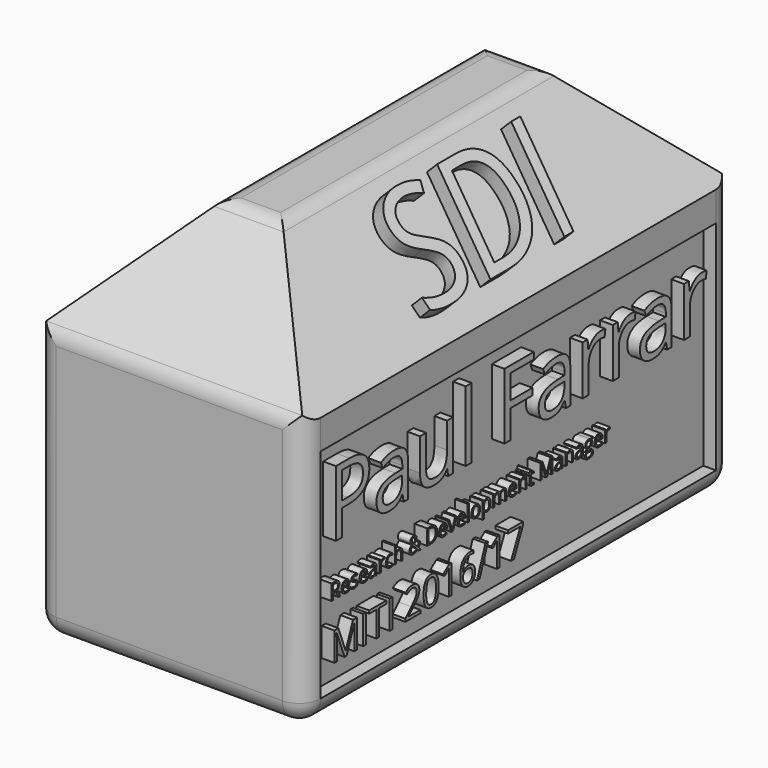
from build123d import *

# Parameters (mm, degrees)
F0_W                    = 63.5
F0_H                    = 63.5
F1_DEPTH                = 63.5
F1_DEPTH_BACK           = 63.5
F2_W                    = 63.5
F2_H                    = 127
F3_DEPTH                = 25
F3_TAPER                = 45
F4_TEXT_SIZE            = 32.8258540119
F5_DEPTH                = 3.4
F6_W                    = 117
F6_H                    = 51.5
F7_DEPTH                = 3
F8_TEXT_SIZE            = 21.8211226941
F8_TEXT_SIZE_2          = 5.1185339948
F8_TEXT_SIZE_3          = 9.4288791944
F9_DEPTH                = 3
F10_W                   = 43.5
F10_H                   = 107
F11_DEPTH               = 60
F12_R                   = 10
F13_R                   = 5
F14_T1_DEPTH            = 53.5
F14_T3_DEPTH            = 71
F14_T5_DEPTH            = 73.8553390593
F14_T7_DEPTH            = 117
F14_T9_DEPTH            = 87.3553390593
F14_T11_DEPTH           = 23.8553390593
F14_S15_W               = 5
F14_S15_H               = 5
F14_T16_DEPTH           = 5
F14_S21_W               = 5
F14_S21_H               = 5
F14_T22_DEPTH           = 5
F14_S27_W               = 5
F14_S27_H               = 5
F14_T28_DEPTH           = 5
F14_S33_W               = 5
F14_S33_H               = 5
F14_T34_DEPTH           = 5
F15_W                   = 33.5
F15_H                   = 87
F16_DEPTH               = 23.2
DRAFT_F16_DRAFTED_ANGLE = 25
F17_R                   = 5


# Not quite as in the source:
# - a fillet or chamfer that OpenCascade refuses, or shapes differently, is made with other operations: its cross-section is extruded or revolved along the edge and cut away or added
# - an extrude with a draft is written as a straight extrude whose walls are then drafted
# - Text() gives the source's letters only with a copy of the font that has no kerning and outlines rounded to 1/6400 em; it was checked with that copy


with BuildPart() as f1:
    # F0 (on Front) → F1 (new body, two sides)
    with BuildSketch(Plane.XZ) as f1_sk:
        Rectangle(F0_W, F0_H)
    extrude(amount=-F1_DEPTH)
    extrude(f1_sk.sketch, amount=F1_DEPTH_BACK)

    # F2 (on face) → F3 (join)
    with BuildSketch(Plane.XY.offset(31.75)):
        Rectangle(F2_W, F2_H)
    extrude(amount=F3_DEPTH, taper=F3_TAPER)

    # F4 (on face) → F5 (join)
    with BuildSketch(Plane(origin=(31.75, 0, 31.75), x_dir=(0, 1, 0), z_dir=(0.7071067812, 0, 0.7071067812))):
        with Locations((-23.613194935, 6.1781886034)):
            Text('SDI', F4_TEXT_SIZE, font='Open Sans', font_style=FontStyle.ITALIC, text_align=(TextAlign.LEFT, TextAlign.BOTTOM))
    extrude(amount=F5_DEPTH)

    # F6 (on face) → F7 (cut)
    with BuildSketch(Plane.YZ.offset(31.75)):
        with Locations((0, -1)):
            Rectangle(F6_W, F6_H)
    extrude(amount=-F7_DEPTH, mode=Mode.SUBTRACT)

    # F8 (on face) → F9 (join)
    with BuildSketch(Plane.YZ.offset(28.75)):
        with Locations((-56.0560356826, 4.2672422715)):
            Text('Paul Farrar', F8_TEXT_SIZE, font='Open Sans', text_align=(TextAlign.LEFT, TextAlign.BOTTOM))
        with Locations((-55.66810444, -7.7586206608)):
            Text('Research & Development Manager', F8_TEXT_SIZE_2, font='Open Sans', text_align=(TextAlign.LEFT, TextAlign.BOTTOM))
        with Locations((-55.28017506, -20.9482768551)):
            Text('MITI 2016/17', F8_TEXT_SIZE_3, font='Open Sans', text_align=(TextAlign.LEFT, TextAlign.BOTTOM))
    extrude(amount=F9_DEPTH)

    # F10 (on face) → F11 (cut)
    with BuildSketch(Plane(origin=(0, 0, -31.75), x_dir=(1, 0, 0), z_dir=(0, 0, -1))):
        Rectangle(F10_W, F10_H)
    extrude(amount=-F11_DEPTH, mode=Mode.SUBTRACT)

    # F12
    f12_edges = [f1.edges().sort_by_distance(p)[0] for p in [
        (0, -53.5, 28.25),
        (0, 53.5, 28.25),
    ]]
    fillet(f12_edges, radius=F12_R)

    # F13
    f13_edges = [f1.edges().sort_by_distance(p)[0] for p in [
        (21.75, 0, 28.25),
        (-21.75, 0, 28.25),
    ]]
    fillet(f13_edges, radius=F13_R)

    # F14: fillet of radius 5 on 14 edges, made by hand

    # F14_s2 → F14_t1 (cut)
    with BuildSketch(Plane.YZ.offset(-26.75)):
        with BuildLine():
            ThreePointArc((58.5, -31.75), (62.0355339059, -30.2855339059), (63.5, -26.75))
            Line((63.5, -26.75), (63.5, -31.75))
            Line((63.5, -31.75), (58.5, -31.75))
        make_face()
        with BuildLine():
            ThreePointArc((-58.5, -31.75), (-62.0355339059, -30.2855339059), (-63.5, -26.75))
            Line((-63.5, -26.75), (-63.5, -31.75))
            Line((-63.5, -31.75), (-58.5, -31.75))
        make_face()
    extrude(amount=F14_T1_DEPTH, mode=Mode.SUBTRACT)

    # F14_s4 → F14_t3 (cut)
    with BuildSketch(Plane.XY.offset(-26.75)):
        with BuildLine():
            ThreePointArc((26.75, 63.5), (30.2855339059, 62.0355339059), (31.75, 58.5))
            Line((31.75, 58.5), (31.75, 63.5))
            Line((31.75, 63.5), (26.75, 63.5))
        make_face()
        with BuildLine():
            ThreePointArc((-26.75, 63.5), (-30.2855339059, 62.0355339059), (-31.75, 58.5))
            Line((-31.75, 58.5), (-31.75, 63.5))
            Line((-31.75, 63.5), (-26.75, 63.5))
        make_face()
        with BuildLine():
            ThreePointArc((31.75, -58.5), (30.2855339059, -62.0355339059), (26.75, -63.5))
            Line((26.75, -63.5), (31.75, -63.5))
            Line((31.75, -63.5), (31.75, -58.5))
        make_face()
        with BuildLine():
            ThreePointArc((-31.75, -58.5), (-30.2855339059, -62.0355339059), (-26.75, -63.5))
            Line((-26.75, -63.5), (-31.75, -63.5))
            Line((-31.75, -63.5), (-31.75, -58.5))
        make_face()
    extrude(amount=F14_T3_DEPTH, mode=Mode.SUBTRACT)

    # F14_s6 → F14_t5 (cut)
    with BuildSketch(Plane.YZ.offset(-36.9276695297)):
        with BuildLine():
            ThreePointArc((63.5, 29.6789321881), (63.1193976626, 31.59234935), (62.0355339059, 33.2144660941))
            Line((62.0355339059, 33.2144660941), (63.5, 31.75))
            Line((63.5, 31.75), (63.5, 29.6789321881))
        make_face()
        with BuildLine():
            ThreePointArc((-63.5, 29.6789321881), (-63.1193976626, 31.59234935), (-62.0355339059, 33.2144660941))
            Line((-62.0355339059, 33.2144660941), (-63.5, 31.75))
            Line((-63.5, 31.75), (-63.5, 29.6789321881))
        make_face()
    extrude(amount=F14_T5_DEPTH, mode=Mode.SUBTRACT)

    # F14_s8 → F14_t7 (cut)
    with BuildSketch(Plane.XZ.offset(-58.5)):
        with BuildLine():
            ThreePointArc((-26.75, -31.75), (-30.2855339059, -30.2855339059), (-31.75, -26.75))
            Line((-31.75, -26.75), (-31.75, -31.75))
            Line((-31.75, -31.75), (-26.75, -31.75))
        make_face()
        with BuildLine():
            ThreePointArc((26.75, -31.75), (30.2855339059, -30.2855339059), (31.75, -26.75))
            Line((31.75, -26.75), (31.75, -31.75))
            Line((31.75, -31.75), (26.75, -31.75))
        make_face()
    extrude(amount=F14_T7_DEPTH, mode=Mode.SUBTRACT)

    # F14_s10 → F14_t9 (cut)
    with BuildSketch(Plane.XZ.offset(-43.6776695297)):
        with BuildLine():
            ThreePointArc((8.2144660941, 55.2855339059), (6.59234935, 56.3693976626), (4.6789321881, 56.75))
            Line((4.6789321881, 56.75), (6.75, 56.75))
            Line((6.75, 56.75), (8.2144660941, 55.2855339059))
        make_face()
        with BuildLine():
            ThreePointArc((-8.2144660941, 55.2855339059), (-6.59234935, 56.3693976626), (-4.6789321881, 56.75))
            Line((-4.6789321881, 56.75), (-6.75, 56.75))
            Line((-6.75, 56.75), (-8.2144660941, 55.2855339059))
        make_face()
    extrude(amount=F14_T9_DEPTH, mode=Mode.SUBTRACT)

    # F14_s12 → F14_t11 (cut)
    with BuildSketch(Plane.YZ.offset(-11.9276695297)):
        with BuildLine():
            ThreePointArc((39.9644660941, 55.2855339059), (38.34234935, 56.3693976626), (36.4289321881, 56.75))
            Line((36.4289321881, 56.75), (38.5, 56.75))
            Line((38.5, 56.75), (39.9644660941, 55.2855339059))
        make_face()
        with BuildLine():
            ThreePointArc((-39.9644660941, 55.2855339059), (-38.34234935, 56.3693976626), (-36.4289321881, 56.75))
            Line((-36.4289321881, 56.75), (-38.5, 56.75))
            Line((-38.5, 56.75), (-39.9644660941, 55.2855339059))
        make_face()
    extrude(amount=F14_T11_DEPTH, mode=Mode.SUBTRACT)


with BuildPart() as f14_tool14:
    # F14_s15 → F14_t16 (new body)
    with BuildSketch(Plane.XY.offset(-26.75)):
        with Locations((-29.25, 61)):
            Rectangle(F14_S15_W, F14_S15_H)
    extrude(amount=-F14_T16_DEPTH)

    # F14_s17 → F14_t18 (revolve, cut)
    with BuildSketch(Plane(origin=(-26.75, 58.5, -26.75), x_dir=(0.7071067812, -0.7071067812, 0), z_dir=(0.7071067812, 0.7071067812, 0))):
        with BuildLine():
            ThreePointArc((0, -5), (5, 0), (0, 5))
            Line((0, 5), (0, -5))
        make_face()
    revolve(axis=Axis((-26.75, 58.5, -26.75), (0, 0, -1)), mode=Mode.SUBTRACT)


with BuildPart() as f1_1:
    add(f1.part)

    # F14_t13: cut F14_tool14
    add(f14_tool14.part, mode=Mode.SUBTRACT)


with BuildPart() as f14_tool20:
    # F14_s21 → F14_t22 (new body)
    with BuildSketch(Plane.XY.offset(-26.75)):
        with Locations((29.25, 61)):
            Rectangle(F14_S21_W, F14_S21_H)
    extrude(amount=-F14_T22_DEPTH)

    # F14_s23 → F14_t24 (revolve, cut)
    with BuildSketch(Plane(origin=(26.75, 58.5, -26.75), x_dir=(-0.7071067812, -0.7071067812, 0), z_dir=(0.7071067812, -0.7071067812, 0))):
        with BuildLine():
            ThreePointArc((0, -5), (5, 0), (0, 5))
            Line((0, 5), (0, -5))
        make_face()
    revolve(axis=Axis((26.75, 58.5, -26.75), (0, 0, -1)), mode=Mode.SUBTRACT)


with BuildPart() as f1_2:
    add(f1_1.part)

    # F14_t19: cut F14_tool20
    add(f14_tool20.part, mode=Mode.SUBTRACT)


with BuildPart() as f14_tool26:
    # F14_s27 → F14_t28 (new body)
    with BuildSketch(Plane.XY.offset(-26.75)):
        with Locations((-29.25, -61)):
            Rectangle(F14_S27_W, F14_S27_H)
    extrude(amount=-F14_T28_DEPTH)

    # F14_s29 → F14_t30 (revolve, cut)
    with BuildSketch(Plane(origin=(-26.75, -58.5, -26.75), x_dir=(0.7071067812, 0.7071067812, 0), z_dir=(-0.7071067812, 0.7071067812, 0))):
        with BuildLine():
            ThreePointArc((0, -5), (5, 0), (0, 5))
            Line((0, 5), (0, -5))
        make_face()
    revolve(axis=Axis((-26.75, -58.5, -26.75), (0, 0, -1)), mode=Mode.SUBTRACT)


with BuildPart() as f1_3:
    add(f1_2.part)

    # F14_t25: cut F14_tool26
    add(f14_tool26.part, mode=Mode.SUBTRACT)


with BuildPart() as f14_tool32:
    # F14_s33 → F14_t34 (new body)
    with BuildSketch(Plane.XY.offset(-26.75)):
        with Locations((29.25, -61)):
            Rectangle(F14_S33_W, F14_S33_H)
    extrude(amount=-F14_T34_DEPTH)

    # F14_s35 → F14_t36 (revolve, cut)
    with BuildSketch(Plane(origin=(26.75, -58.5, -26.75), x_dir=(-0.7071067812, 0.7071067812, 0), z_dir=(-0.7071067812, -0.7071067812, 0))):
        with BuildLine():
            ThreePointArc((0, -5), (5, 0), (0, 5))
            Line((0, 5), (0, -5))
        make_face()
    revolve(axis=Axis((26.75, -58.5, -26.75), (0, 0, -1)), mode=Mode.SUBTRACT)


with BuildPart() as f1_4:
    add(f1_3.part)

    # F14_t31: cut F14_tool32
    add(f14_tool32.part, mode=Mode.SUBTRACT)


with BuildPart() as f16_drafted:
    # F15 (on face) → F16 (new body)
    with BuildSketch(Plane(origin=(0, 0, 28.25), x_dir=(1, 0, 0), z_dir=(0, 0, -1))):
        Rectangle(F15_W, F15_H)
    extrude(amount=-F16_DEPTH)

    # draft_F16_drafted
    draft_f16_drafted_walls = [f16_drafted.faces().sort_by_distance(p)[0] for p in [
        (16.75, 0, 43.7166666667),
        (0, -43.5, 43.7166666667),
        (-16.75, 0, 43.7166666667),
        (0, 43.5, 43.7166666667),
    ]]
    draft(draft_f16_drafted_walls, neutral_plane=Plane.XY.offset(28.25), angle=DRAFT_F16_DRAFTED_ANGLE)


with BuildPart() as f1_5:
    add(f1_4.part)

    # join_F16_drafted: cut F16_drafted
    add(f16_drafted.part, mode=Mode.SUBTRACT)

    # F17
    f17_edges = [f1_5.edges().sort_by_distance(p)[0] for p in [
        (5.931662, 0, 51.45),
        (0, -32.681662, 51.45),
        (-5.931662, 0, 51.45),
        (0, 32.681662, 51.45),
    ]]
    fillet(f17_edges, radius=F17_R)


solid = f1_5.part
